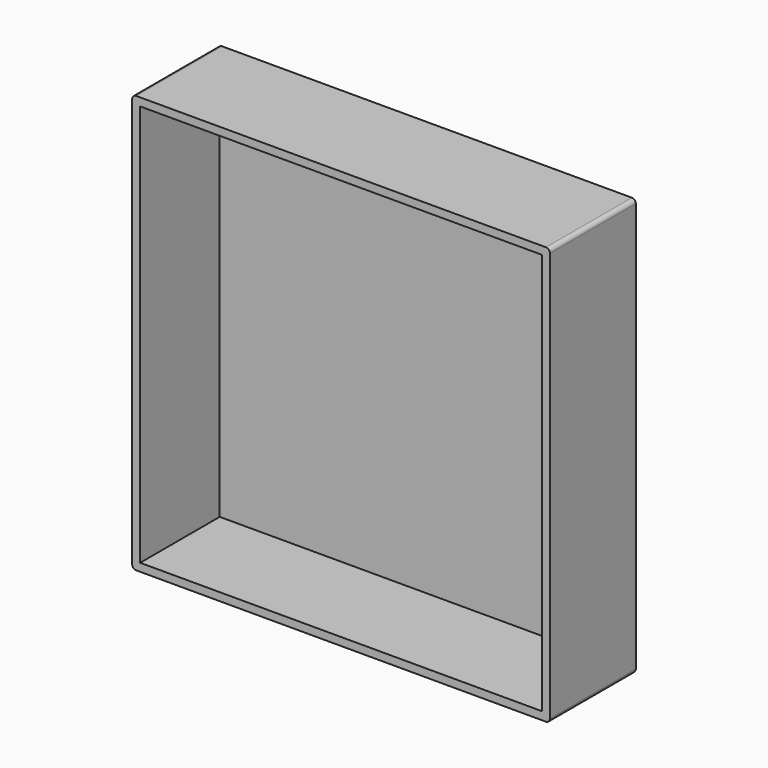
from build123d import *

# Parameters (mm, degrees)
F0_W         = 105
F0_H         = 105
F1_DEPTH     = 27
F2_T         = -2
F3_TEXT_SIZE = 18.1321882539
F4_DEPTH     = 1.5
F5_R         = 1


# Not quite as in the source:
# - Text() gives the source's letters only with a copy of the font that has no kerning and outlines rounded to 1/6400 em; it was checked with that copy


with BuildPart() as f1:
    # F0 (on Front) → F1 (new body)
    with BuildSketch(Plane.XZ):
        with Locations((14.5822350383, 5.4051420137)):
            Rectangle(F0_W, F0_H)
    extrude(amount=F1_DEPTH)

    # F2
    f2_openings = [f1.faces().sort_by_distance(p)[0] for p in [
        (14.582235, -27, 5.405142),
    ]]
    offset(amount=F2_T, openings=f2_openings)

    # F3 (on face) → F4 (cut)
    with BuildSketch(Plane(origin=(0, 0, 0), x_dir=(-1, 0, 0), z_dir=(0, 1, 0))):
        with Locations((-46.2876409292, 32.7588319778)):
            Text('HKYau', F3_TEXT_SIZE, font='Open Sans', text_align=(TextAlign.LEFT, TextAlign.BOTTOM))
    extrude(amount=-F4_DEPTH, mode=Mode.SUBTRACT)

    # F5
    f5_edges = [f1.edges().sort_by_distance(p)[0] for p in [
        (67.082235, -13.5, -47.094858),
        (-37.917765, -13.5, -47.094858),
        (67.082235, -13.5, 57.905142),
        (-37.917765, -13.5, 57.905142),
    ]]
    fillet(f5_edges, radius=F5_R)


solid = f1.part
